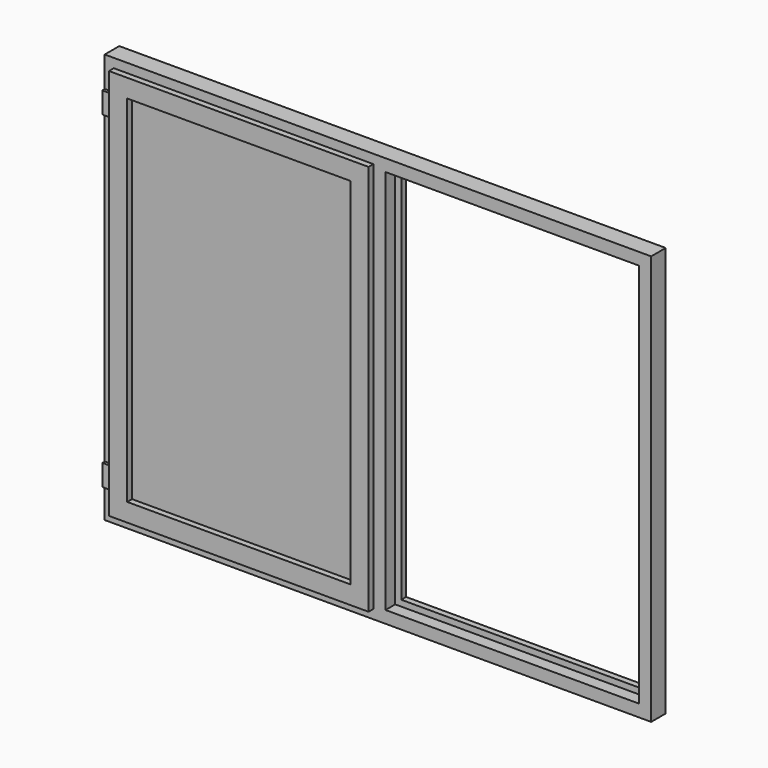
from build123d import *

# Parameters (mm, degrees)
F0_W          = 1800
F0_H          = 1350
F1_DEPTH      = 40
F0_W_2        = 50
F0_H_2        = 1230
F0_W_3        = 20
F0_H_3        = 20
F2_DEPTH      = 20
F3_DEPTH      = 40
F3_DEPTH_BACK = 20
F4_W          = 835
F4_H          = 1270
F4_W_2        = 735
F4_H_2        = 1170
F5_DEPTH      = 40
F6_DEPTH      = 20
F7_DEPTH      = 10
F4_W_3        = 30
F4_H_3        = 70
F8_DEPTH      = 10


with BuildPart() as f1:
    # F0 (on Front) → F1 (new body)
    with BuildSketch(Plane.XZ):
        Rectangle(F0_W, F0_H)
        Polygon((-860, -635), (-860, 635), (-25, 635), (25, 635), (860, 635), (860, -635), (25, -635), (-25, -635), align=None, mode=Mode.SUBTRACT)
    extrude(amount=F1_DEPTH)

    # F0 (on Front) → F2 (join)
    with BuildSketch(Plane.XZ):
        Rectangle(F0_W, F0_H)
        Polygon((-860, -635), (-860, 635), (-25, 635), (25, 635), (860, 635), (860, -635), (25, -635), (-25, -635), align=None, mode=Mode.SUBTRACT)
        Rectangle(F0_W_2, F0_H_2)
        Polygon((-25, 635), (-860, 635), (-860, -635), (-25, -635), (-25, -615), (-45, -615), (-840, -615), (-840, 615), (-45, 615), (-25, 615), align=None)
        Polygon((860, 635), (25, 635), (25, 615), (45, 615), (840, 615), (840, -615), (45, -615), (25, -615), (25, -635), (860, -635), align=None)
        with Locations((35, 0)):
            Rectangle(F0_W_3, F0_H_2)
        with Locations((-35, 0)):
            Rectangle(F0_W_3, F0_H_2)
        with Locations((0, -625)):
            Rectangle(F0_W_2, F0_H_3)
        with Locations((0, 625)):
            Rectangle(F0_W_2, F0_H_3)
    extrude(amount=-F2_DEPTH)

    # F0 (on Front) → F3 (join, two sides)
    with BuildSketch(Plane.XZ) as f3_sk:
        Rectangle(F0_W_2, F0_H_2)
        with Locations((0, 625)):
            Rectangle(F0_W_2, F0_H_3)
        with Locations((0, -625)):
            Rectangle(F0_W_2, F0_H_3)
    extrude(amount=F3_DEPTH)
    extrude(f3_sk.sketch, amount=-F3_DEPTH_BACK)


with BuildPart() as f5:
    # F4 (on face) → F5 (new body, through all)
    with BuildSketch(Plane.XZ.offset(40)):
        with Locations((-442.5, 0)):
            Rectangle(F4_W, F4_H)
        with Locations((-442.5, 0)):
            Rectangle(F4_W_2, F4_H_2, mode=Mode.SUBTRACT)
    extrude(amount=-F5_DEPTH)

    # F4 (on face) → F6 (join)
    with BuildSketch(Plane.XZ.offset(40)):
        Polygon((-870, -575), (-870, -645), (-15, -645), (-15, 645), (-870, 645), (-870, 575), (-870, 505), (-870, -505), align=None)
        with Locations((-442.5, 0)):
            Rectangle(F4_W, F4_H, mode=Mode.SUBTRACT)
        with Locations((-442.5, 0)):
            Rectangle(F4_W, F4_H)
        with Locations((-442.5, 0)):
            Rectangle(F4_W_2, F4_H_2, mode=Mode.SUBTRACT)
    extrude(amount=F6_DEPTH)

    # F4 (on face) → F8 (join)
    with BuildSketch(Plane.XZ.offset(40)):
        with Locations((-885, 540)):
            Rectangle(F4_W_3, F4_H_3)
        with Locations((-885, -540)):
            Rectangle(F4_W_3, F4_H_3)
    extrude(amount=F8_DEPTH)


with BuildPart() as f7:
    # F4 (on face) → F7 (new body)
    with BuildSketch(Plane.XZ.offset(40)):
        with Locations((-442.5, 0)):
            Rectangle(F4_W_2, F4_H_2)
    extrude(amount=-F7_DEPTH)


solid = Compound([f1.part, f5.part, f7.part])
